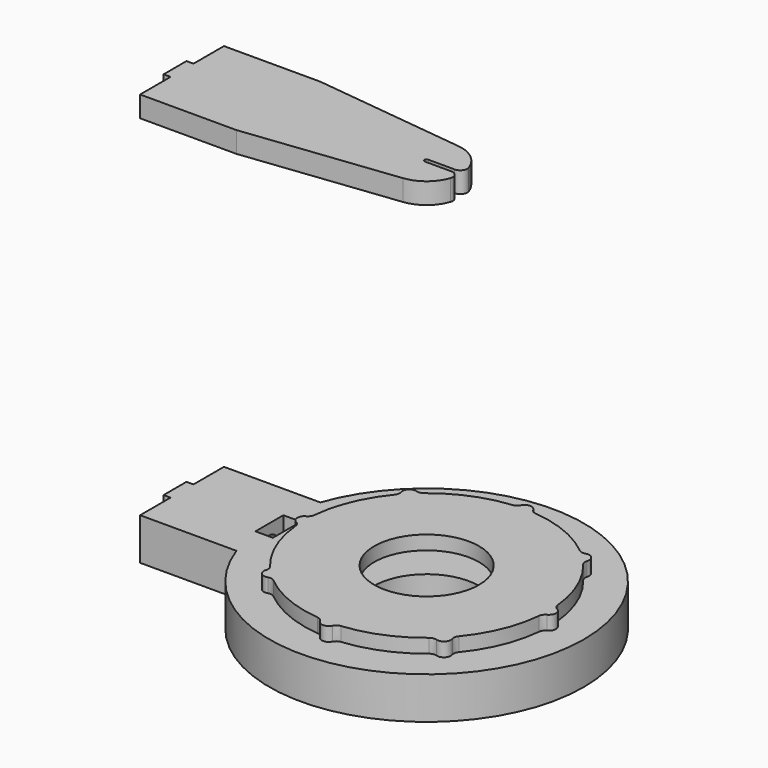
from build123d import *

# Parameters (mm, degrees)
F0_R            = 35
F0_R_2          = 15
F1_DEPTH        = 6
F2_DEPTH        = 12
F3_R            = 2
F4_DEPTH        = 6
F4_COPIES_COUNT = 8
F5_R            = 2
F6_W            = 5
F6_H            = 10
F7_DEPTH        = 12
F8_W            = 8.2
F8_H            = 12
F9_DEPTH        = 2
F10_R           = 15
F11_DEPTH       = 4
F14_DEPTH       = 6
F15_R           = 3
F16_DEPTH       = 27


# Not quite as in the source:
# - a pattern or mirror of a feature is missing from the dataset's text; its kind, count and spacing are read off the source's solid


with BuildPart() as f1:
    # F0 (on Top) → F1 (new body)
    with BuildSketch(Plane.XY):
        Circle(F0_R)
        Circle(F0_R_2, mode=Mode.SUBTRACT)
    extrude(amount=F1_DEPTH)

    # F0 (on Top) → F2 (join)
    with BuildSketch(Plane.XY):
        with BuildLine():
            ThreePointArc((-42.4264068712, -15), (7.6095890427, -44.3519351844), (45, 0))
            ThreePointArc((45, 0), (7.6095890427, 44.3519351844), (-42.4264068712, 15))
            ThreePointArc((-42.4264068712, 15), (-45, 0), (-42.4264068712, -15))
        make_face()
        Circle(F0_R, mode=Mode.SUBTRACT)
        with BuildLine():
            ThreePointArc((-42.4264068712, -15), (-45, 0), (-42.4264068712, 15))
            Line((-42.4264068712, 15), (-70, 15))
            Line((-70, 15), (-70, -15))
            Line((-70, -15), (-42.4264068712, -15))
        make_face()
    extrude(amount=F2_DEPTH)

    # F3 (on face) → F4 (cut, through all)
    with BuildSketch(Plane.XY.offset(12)):
        with Locations((0, 35)):
            Circle(F3_R)
    f4 = extrude(amount=-F4_DEPTH, mode=Mode.SUBTRACT)

    # F4_copies: F4 ×8 about axis
    f4_copies_axis = Axis((0, 0, 0), (0, 0, 1))
    for i in range(1, F4_COPIES_COUNT):
        add(f4.rotate(f4_copies_axis, i * 360 / F4_COPIES_COUNT), mode=Mode.SUBTRACT)

    # F5
    f5_edges = [f1.edges().sort_by_distance(p)[0] for p in [
        (1.999184, 34.942857, 9),
        (-1.999184, 34.942857, 9),
        (23.294695, 26.121967, 9),
        (26.121967, 23.294695, 9),
        (34.942857, 1.999184, 9),
        (34.942857, -1.999184, 9),
        (26.121967, -23.294695, 9),
        (23.294695, -26.121967, 9),
        (1.999184, -34.942857, 9),
        (-1.999184, -34.942857, 9),
        (-23.294695, -26.121967, 9),
        (-26.121967, -23.294695, 9),
        (-34.942857, -1.999184, 9),
        (-34.942857, 1.999184, 9),
        (-26.121967, 23.294695, 9),
        (-23.294695, 26.121967, 9),
    ]]
    fillet(f5_edges, radius=F5_R)

    # F6 (on face) → F7 (cut, through all)
    with BuildSketch(Plane.XY.offset(12)):
        with Locations((-42.5, 0)):
            Rectangle(F6_W, F6_H)
    extrude(amount=-F7_DEPTH, mode=Mode.SUBTRACT)

    # F8 (on face) → F9 (join)
    with BuildSketch(Plane(origin=(-70, 0, 0), x_dir=(0, -1, 0), z_dir=(-1, 0, 0))):
        with Locations((0, 6)):
            Rectangle(F8_W, F8_H)
    extrude(amount=F9_DEPTH)

    # F15 (on face) → F16 (cut, through all)
    with BuildSketch(Plane(origin=(-72, 0, 0), x_dir=(0, -1, 0), z_dir=(-1, 0, 0))):
        with Locations((0, 6)):
            Circle(F15_R)
    extrude(amount=-F16_DEPTH, mode=Mode.SUBTRACT)


with BuildPart() as f11:
    # F10 (on face) → F11 (new body)
    with BuildSketch(Plane.XY.offset(12)):
        with BuildLine():
            add(Edge.make_bspline(
                [(-24.1374429299, 26.6530270102), (-24.0459440301, 26.623655026), (-23.9514078399, 26.5993696847), (-23.854346504, 26.5806739313), (-23.7554183378, 26.5679730914), (-23.5549954164, 26.5549969713), (-23.4534922591, 26.5547609879), (-23.3516036224, 26.561020377), (-23.2501506832, 26.573824975), (-23.0496949529, 26.6122187008), (-22.9506907158, 26.6378081055), (-22.853700131, 26.66964049), (-22.7594678434, 26.7073661126), (-22.5780242256, 26.7934819687), (-22.4907905674, 26.8418387912), (-22.4075067936, 26.8950764391), (-22.3286348574, 26.9525750193), (-22.2544648145, 27.0136779395)],
                knots=[0, 0, 0, 0, 0, 0, 0.2496046148, 0.2496046148, 0.2496046148, 0.2496046148, 0.5, 0.5, 0.5, 0.5, 0.7503953852, 0.7503953852, 0.7503953852, 0.7503953852, 1, 1, 1, 1, 1, 1], degree=5))
            ThreePointArc((-24.1374429299, 26.6530270102), (-26.1629509039, 26.1629509039), (-26.6530270102, 24.1374429299))
            add(Edge.make_bspline(
                [(-27.0136779395, 22.2544648145), (-26.9525750193, 22.3286348574), (-26.8950764391, 22.4075067936), (-26.8418387912, 22.4907905674), (-26.7934819687, 22.5780242256), (-26.7073661126, 22.7594678434), (-26.66964049, 22.853700131), (-26.6378081055, 22.9506907158), (-26.6122187008, 23.0496949529), (-26.573824975, 23.2501506832), (-26.561020377, 23.3516036224), (-26.5547609879, 23.4534922591), (-26.5549969713, 23.5549954164), (-26.5679730914, 23.7554183378), (-26.5806739313, 23.854346504), (-26.5993696847, 23.9514078399), (-26.623655026, 24.0459440301), (-26.6530270102, 24.1374429299)],
                knots=[0, 0, 0, 0, 0, 0, 0.2496046148, 0.2496046148, 0.2496046148, 0.2496046148, 0.5, 0.5, 0.5, 0.5, 0.7503953852, 0.7503953852, 0.7503953852, 0.7503953852, 1, 1, 1, 1, 1, 1], degree=5))
            ThreePointArc((-27.0136779395, 22.2544648145), (-32.3357836379, 13.3939201328), (-34.8378378378, 3.3652718738))
            add(Edge.make_bspline(
                [(-35.9142857143, 1.7787865619), (-35.8288170926, 1.8227169251), (-35.7447975819, 1.8723917768), (-35.6629449591, 1.9278046116), (-35.5840113319, 1.9887765388), (-35.4331154226, 2.1213214431), (-35.3611749863, 2.1929281484), (-35.2935548968, 2.2694003508), (-35.2308710536, 2.3501926302), (-35.1162759112, 2.5190847003), (-35.0643637854, 2.6071857093), (-35.0182899801, 2.6982773045), (-34.9783337341, 2.7915856376), (-34.9109268274, 2.9807787559), (-34.8834367532, 3.0766557043), (-34.8621909339, 3.1731909274), (-34.8470776888, 3.2696194443), (-34.8378378378, 3.3652718738)],
                knots=[0, 0, 0, 0, 0, 0, 0.2496046148, 0.2496046148, 0.2496046148, 0.2496046148, 0.5, 0.5, 0.5, 0.5, 0.7503953852, 0.7503953852, 0.7503953852, 0.7503953852, 1, 1, 1, 1, 1, 1], degree=5))
            ThreePointArc((-35.9142857143, 1.7787865619), (-37, 0), (-35.9142857143, -1.7787865619))
            add(Edge.make_bspline(
                [(-34.8378378378, -3.3652718738), (-34.8470776888, -3.2696194443), (-34.8621909339, -3.1731909274), (-34.8834367532, -3.0766557043), (-34.9109268274, -2.9807787559), (-34.9783337341, -2.7915856376), (-35.0182899801, -2.6982773045), (-35.0643637854, -2.6071857093), (-35.1162759112, -2.5190847003), (-35.2308710536, -2.3501926302), (-35.2935548968, -2.2694003508), (-35.3611749863, -2.1929281484), (-35.4331154226, -2.1213214431), (-35.5840113319, -1.9887765388), (-35.6629449591, -1.9278046116), (-35.7447975819, -1.8723917768), (-35.8288170926, -1.8227169251), (-35.9142857143, -1.7787865619)],
                knots=[0, 0, 0, 0, 0, 0, 0.2496046148, 0.2496046148, 0.2496046148, 0.2496046148, 0.5, 0.5, 0.5, 0.5, 0.7503953852, 0.7503953852, 0.7503953852, 0.7503953852, 1, 1, 1, 1, 1, 1], degree=5))
            ThreePointArc((-34.8378378378, -3.3652718738), (-32.3357836379, -13.3939201328), (-27.0136779395, -22.2544648145))
            add(Edge.make_bspline(
                [(-26.6530270102, -24.1374429299), (-26.623655026, -24.0459440301), (-26.5993696847, -23.9514078399), (-26.5806739313, -23.854346504), (-26.5679730914, -23.7554183378), (-26.5549969713, -23.5549954164), (-26.5547609879, -23.4534922591), (-26.561020377, -23.3516036224), (-26.573824975, -23.2501506832), (-26.6122187008, -23.0496949529), (-26.6378081055, -22.9506907158), (-26.66964049, -22.853700131), (-26.7073661126, -22.7594678434), (-26.7934819687, -22.5780242256), (-26.8418387912, -22.4907905674), (-26.8950764391, -22.4075067936), (-26.9525750193, -22.3286348574), (-27.0136779395, -22.2544648145)],
                knots=[0, 0, 0, 0, 0, 0, 0.2496046148, 0.2496046148, 0.2496046148, 0.2496046148, 0.5, 0.5, 0.5, 0.5, 0.7503953852, 0.7503953852, 0.7503953852, 0.7503953852, 1, 1, 1, 1, 1, 1], degree=5))
            ThreePointArc((-26.6530270102, -24.1374429299), (-26.1629509039, -26.1629509039), (-24.1374429299, -26.6530270102))
            add(Edge.make_bspline(
                [(-22.2544648145, -27.0136779395), (-22.3286348574, -26.9525750193), (-22.4075067936, -26.8950764391), (-22.4907905674, -26.8418387912), (-22.5780242256, -26.7934819687), (-22.7594678434, -26.7073661126), (-22.853700131, -26.66964049), (-22.9506907158, -26.6378081055), (-23.0496949529, -26.6122187008), (-23.2501506832, -26.573824975), (-23.3516036224, -26.561020377), (-23.4534922591, -26.5547609879), (-23.5549954164, -26.5549969713), (-23.7554183378, -26.5679730914), (-23.854346504, -26.5806739313), (-23.9514078399, -26.5993696847), (-24.0459440301, -26.623655026), (-24.1374429299, -26.6530270102)],
                knots=[0, 0, 0, 0, 0, 0, 0.2496046148, 0.2496046148, 0.2496046148, 0.2496046148, 0.5, 0.5, 0.5, 0.5, 0.7503953852, 0.7503953852, 0.7503953852, 0.7503953852, 1, 1, 1, 1, 1, 1], degree=5))
            ThreePointArc((-22.2544648145, -27.0136779395), (-13.3939201328, -32.3357836379), (-3.3652718738, -34.8378378378))
            add(Edge.make_bspline(
                [(-1.7787865619, -35.9142857143), (-1.8227169251, -35.8288170926), (-1.8723917768, -35.7447975819), (-1.9278046116, -35.6629449591), (-1.9887765388, -35.5840113319), (-2.1213214431, -35.4331154226), (-2.1929281484, -35.3611749863), (-2.2694003508, -35.2935548968), (-2.3501926302, -35.2308710536), (-2.5190847003, -35.1162759112), (-2.6071857093, -35.0643637854), (-2.6982773045, -35.0182899801), (-2.7915856376, -34.9783337341), (-2.9807787559, -34.9109268274), (-3.0766557043, -34.8834367532), (-3.1731909274, -34.8621909339), (-3.2696194443, -34.8470776888), (-3.3652718738, -34.8378378378)],
                knots=[0, 0, 0, 0, 0, 0, 0.2496046148, 0.2496046148, 0.2496046148, 0.2496046148, 0.5, 0.5, 0.5, 0.5, 0.7503953852, 0.7503953852, 0.7503953852, 0.7503953852, 1, 1, 1, 1, 1, 1], degree=5))
            ThreePointArc((-1.7787865619, -35.9142857143), (0, -37), (1.7787865619, -35.9142857143))
            add(Edge.make_bspline(
                [(3.3652718738, -34.8378378378), (3.2696194443, -34.8470776888), (3.1731909274, -34.8621909339), (3.0766557043, -34.8834367532), (2.9807787559, -34.9109268274), (2.7915856376, -34.9783337341), (2.6982773045, -35.0182899801), (2.6071857093, -35.0643637854), (2.5190847003, -35.1162759112), (2.3501926302, -35.2308710536), (2.2694003508, -35.2935548968), (2.1929281484, -35.3611749863), (2.1213214431, -35.4331154226), (1.9887765388, -35.5840113319), (1.9278046116, -35.6629449591), (1.8723917768, -35.7447975819), (1.8227169251, -35.8288170926), (1.7787865619, -35.9142857143)],
                knots=[0, 0, 0, 0, 0, 0, 0.2496046148, 0.2496046148, 0.2496046148, 0.2496046148, 0.5, 0.5, 0.5, 0.5, 0.7503953852, 0.7503953852, 0.7503953852, 0.7503953852, 1, 1, 1, 1, 1, 1], degree=5))
            ThreePointArc((3.3652718738, -34.8378378378), (13.3939201328, -32.3357836379), (22.2544648145, -27.0136779395))
            add(Edge.make_bspline(
                [(24.1374429299, -26.6530270102), (24.0459440301, -26.623655026), (23.9514078399, -26.5993696847), (23.854346504, -26.5806739313), (23.7554183378, -26.5679730914), (23.5549954164, -26.5549969713), (23.4534922591, -26.5547609879), (23.3516036224, -26.561020377), (23.2501506832, -26.573824975), (23.0496949529, -26.6122187008), (22.9506907158, -26.6378081055), (22.853700131, -26.66964049), (22.7594678434, -26.7073661126), (22.5780242256, -26.7934819687), (22.4907905674, -26.8418387912), (22.4075067936, -26.8950764391), (22.3286348574, -26.9525750193), (22.2544648145, -27.0136779395)],
                knots=[0, 0, 0, 0, 0, 0, 0.2496046148, 0.2496046148, 0.2496046148, 0.2496046148, 0.5, 0.5, 0.5, 0.5, 0.7503953852, 0.7503953852, 0.7503953852, 0.7503953852, 1, 1, 1, 1, 1, 1], degree=5))
            ThreePointArc((24.1374429299, -26.6530270102), (26.1629509039, -26.1629509039), (26.6530270102, -24.1374429299))
            add(Edge.make_bspline(
                [(27.0136779395, -22.2544648145), (26.9525750193, -22.3286348574), (26.8950764391, -22.4075067936), (26.8418387912, -22.4907905674), (26.7934819687, -22.5780242256), (26.7073661126, -22.7594678434), (26.66964049, -22.853700131), (26.6378081055, -22.9506907158), (26.6122187008, -23.0496949529), (26.573824975, -23.2501506832), (26.561020377, -23.3516036224), (26.5547609879, -23.4534922591), (26.5549969713, -23.5549954164), (26.5679730914, -23.7554183378), (26.5806739313, -23.854346504), (26.5993696847, -23.9514078399), (26.623655026, -24.0459440301), (26.6530270102, -24.1374429299)],
                knots=[0, 0, 0, 0, 0, 0, 0.2496046148, 0.2496046148, 0.2496046148, 0.2496046148, 0.5, 0.5, 0.5, 0.5, 0.7503953852, 0.7503953852, 0.7503953852, 0.7503953852, 1, 1, 1, 1, 1, 1], degree=5))
            ThreePointArc((27.0136779395, -22.2544648145), (32.3357836379, -13.3939201328), (34.8378378378, -3.3652718738))
            add(Edge.make_bspline(
                [(35.9142857143, -1.7787865619), (35.8288170926, -1.8227169251), (35.7447975819, -1.8723917768), (35.6629449591, -1.9278046116), (35.5840113319, -1.9887765388), (35.4331154226, -2.1213214431), (35.3611749863, -2.1929281484), (35.2935548968, -2.2694003508), (35.2308710536, -2.3501926302), (35.1162759112, -2.5190847003), (35.0643637854, -2.6071857093), (35.0182899801, -2.6982773045), (34.9783337341, -2.7915856376), (34.9109268274, -2.9807787559), (34.8834367532, -3.0766557043), (34.8621909339, -3.1731909274), (34.8470776888, -3.2696194443), (34.8378378378, -3.3652718738)],
                knots=[0, 0, 0, 0, 0, 0, 0.2496046148, 0.2496046148, 0.2496046148, 0.2496046148, 0.5, 0.5, 0.5, 0.5, 0.7503953852, 0.7503953852, 0.7503953852, 0.7503953852, 1, 1, 1, 1, 1, 1], degree=5))
            ThreePointArc((35.9142857143, -1.7787865619), (37, 0), (35.9142857143, 1.7787865619))
            add(Edge.make_bspline(
                [(34.8378378378, 3.3652718738), (34.8470776888, 3.2696194443), (34.8621909339, 3.1731909274), (34.8834367532, 3.0766557043), (34.9109268274, 2.9807787559), (34.9783337341, 2.7915856376), (35.0182899801, 2.6982773045), (35.0643637854, 2.6071857093), (35.1162759112, 2.5190847003), (35.2308710536, 2.3501926302), (35.2935548968, 2.2694003508), (35.3611749863, 2.1929281484), (35.4331154226, 2.1213214431), (35.5840113319, 1.9887765388), (35.6629449591, 1.9278046116), (35.7447975819, 1.8723917768), (35.8288170926, 1.8227169251), (35.9142857143, 1.7787865619)],
                knots=[0, 0, 0, 0, 0, 0, 0.2496046148, 0.2496046148, 0.2496046148, 0.2496046148, 0.5, 0.5, 0.5, 0.5, 0.7503953852, 0.7503953852, 0.7503953852, 0.7503953852, 1, 1, 1, 1, 1, 1], degree=5))
            ThreePointArc((34.8378378378, 3.3652718738), (32.3357836379, 13.3939201328), (27.0136779395, 22.2544648145))
            add(Edge.make_bspline(
                [(26.6530270102, 24.1374429299), (26.623655026, 24.0459440301), (26.5993696847, 23.9514078399), (26.5806739313, 23.854346504), (26.5679730914, 23.7554183378), (26.5549969713, 23.5549954164), (26.5547609879, 23.4534922591), (26.561020377, 23.3516036224), (26.573824975, 23.2501506832), (26.6122187008, 23.0496949529), (26.6378081055, 22.9506907158), (26.66964049, 22.853700131), (26.7073661126, 22.7594678434), (26.7934819687, 22.5780242256), (26.8418387912, 22.4907905674), (26.8950764391, 22.4075067936), (26.9525750193, 22.3286348574), (27.0136779395, 22.2544648145)],
                knots=[0, 0, 0, 0, 0, 0, 0.2496046148, 0.2496046148, 0.2496046148, 0.2496046148, 0.5, 0.5, 0.5, 0.5, 0.7503953852, 0.7503953852, 0.7503953852, 0.7503953852, 1, 1, 1, 1, 1, 1], degree=5))
            ThreePointArc((26.6530270102, 24.1374429299), (26.1629509039, 26.1629509039), (24.1374429299, 26.6530270102))
            add(Edge.make_bspline(
                [(22.2544648145, 27.0136779395), (22.3286348574, 26.9525750193), (22.4075067936, 26.8950764391), (22.4907905674, 26.8418387912), (22.5780242256, 26.7934819687), (22.7594678434, 26.7073661126), (22.853700131, 26.66964049), (22.9506907158, 26.6378081055), (23.0496949529, 26.6122187008), (23.2501506832, 26.573824975), (23.3516036224, 26.561020377), (23.4534922591, 26.5547609879), (23.5549954164, 26.5549969713), (23.7554183378, 26.5679730914), (23.854346504, 26.5806739313), (23.9514078399, 26.5993696847), (24.0459440301, 26.623655026), (24.1374429299, 26.6530270102)],
                knots=[0, 0, 0, 0, 0, 0, 0.2496046148, 0.2496046148, 0.2496046148, 0.2496046148, 0.5, 0.5, 0.5, 0.5, 0.7503953852, 0.7503953852, 0.7503953852, 0.7503953852, 1, 1, 1, 1, 1, 1], degree=5))
            ThreePointArc((22.2544648145, 27.0136779395), (13.3939201328, 32.3357836379), (3.3652718738, 34.8378378378))
            add(Edge.make_bspline(
                [(3.3652718738, 34.8378378378), (3.2696194443, 34.8470776888), (3.1731909274, 34.8621909339), (3.0766557043, 34.8834367532), (2.9807787559, 34.9109268274), (2.7915856376, 34.9783337341), (2.6982773045, 35.0182899801), (2.6071857093, 35.0643637854), (2.5190847003, 35.1162759112), (2.3501926302, 35.2308710536), (2.2694003508, 35.2935548968), (2.1929281484, 35.3611749863), (2.1213214431, 35.4331154226), (1.9887765388, 35.5840113319), (1.9278046116, 35.6629449591), (1.8723917768, 35.7447975819), (1.8227169251, 35.8288170926), (1.7787865619, 35.9142857143)],
                knots=[0, 0, 0, 0, 0, 0, 0.2496046148, 0.2496046148, 0.2496046148, 0.2496046148, 0.5, 0.5, 0.5, 0.5, 0.7503953852, 0.7503953852, 0.7503953852, 0.7503953852, 1, 1, 1, 1, 1, 1], degree=5))
            ThreePointArc((1.7787865619, 35.9142857143), (0, 37), (-1.7787865619, 35.9142857143))
            add(Edge.make_bspline(
                [(-3.3652718738, 34.8378378378), (-3.2696194443, 34.8470776888), (-3.1731909274, 34.8621909339), (-3.0766557043, 34.8834367532), (-2.9807787559, 34.9109268274), (-2.7915856376, 34.9783337341), (-2.6982773045, 35.0182899801), (-2.6071857093, 35.0643637854), (-2.5190847003, 35.1162759112), (-2.3501926302, 35.2308710536), (-2.2694003508, 35.2935548968), (-2.1929281484, 35.3611749863), (-2.1213214431, 35.4331154226), (-1.9887765388, 35.5840113319), (-1.9278046116, 35.6629449591), (-1.8723917768, 35.7447975819), (-1.8227169251, 35.8288170926), (-1.7787865619, 35.9142857143)],
                knots=[0, 0, 0, 0, 0, 0, 0.2496046148, 0.2496046148, 0.2496046148, 0.2496046148, 0.5, 0.5, 0.5, 0.5, 0.7503953852, 0.7503953852, 0.7503953852, 0.7503953852, 1, 1, 1, 1, 1, 1], degree=5))
            ThreePointArc((-3.3652718738, 34.8378378378), (-13.3939201328, 32.3357836379), (-22.2544648145, 27.0136779395))
        make_face()
        Circle(F10_R, mode=Mode.SUBTRACT)
    extrude(amount=F11_DEPTH)


with BuildPart() as f14:
    # F13 (on offset) → F14 (new body)
    with BuildSketch(Plane.XY.offset(112)):
        with BuildLine():
            ThreePointArc((1.1548556066, -9.9330915896), (-10, 0), (1.1548556066, 9.9330915896))
            Line((1.1548556066, 9.9330915896), (-42.4264068712, 15))
            Line((-42.4264068712, 15), (-70, 15))
            Line((-70, 15), (-70, 4.1))
            Line((-70, 4.1), (-72, 4.1))
            Line((-72, 4.1), (-72, -4.1))
            Line((-72, -4.1), (-70, -4.1))
            Line((-70, -4.1), (-70, -15))
            Line((-70, -15), (-42.4264068712, -15))
            Line((-42.4264068712, -15), (1.1548556066, -9.9330915896))
        make_face()
        with BuildLine():
            ThreePointArc((0, -0.6), (-0.6, 0), (0, 0.6))
            Line((0, 0.6), (7.5657121278, 0.6))
            ThreePointArc((7.5657121278, 0.6), (9.1935941874, 1.4381049961), (9.4571401597, 3.25))
            ThreePointArc((9.4571401597, 3.25), (6.2705296295, 7.7897662459), (1.1548556066, 9.9330915896))
            ThreePointArc((1.1548556066, 9.9330915896), (-10, 0), (1.1548556066, -9.9330915896))
            ThreePointArc((1.1548556066, -9.9330915896), (6.2705296295, -7.7897662459), (9.4571401597, -3.25))
            ThreePointArc((9.4571401597, -3.25), (9.1935941874, -1.4381049961), (7.5657121278, -0.6))
            Line((7.5657121278, -0.6), (0, -0.6))
        make_face()
    extrude(amount=F14_DEPTH)


solid = Compound([f1.part, f11.part, f14.part])
